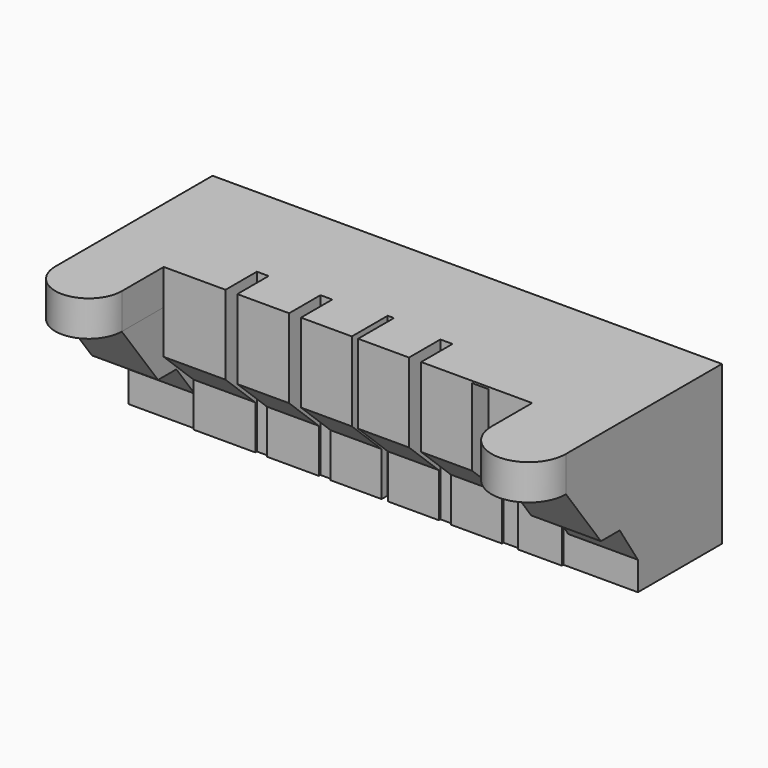
from build123d import *

# Parameters (mm, degrees)
F0_W      = 154.4681414962
F0_H      = 32.4599891901
F1_DEPTH  = 48.0146426708
F2_W      = 11.2775340676
F2_H      = 24.0073213354
F3_DEPTH  = 154.6795647591
F4_W      = 20.4018931836
F4_H      = 24.0073213354
F4_W_2    = 3.5617277026
F4_W_3    = 3.5835206509
F4_W_4    = 3.6845356226
F4_W_5    = 4.9127191305
F4_W_6    = 22.562906146
F4_H_2    = 23.4004920349
F5_DEPTH  = 11.8805598468
F7_DEPTH  = 10.7736643404
F9_DEPTH  = 20.0494788587
F11_DEPTH = 21.1268346757
F12_W     = 1.8992722034
F12_H     = 24.0073213354
F13_DEPTH = 13.5909728706


with BuildPart() as f1:
    # F0 (on Top) → F1 (new body)
    with BuildSketch(Plane.XY):
        with Locations((3.7253e-06, -0.5876496434)):
            Rectangle(F0_W, F0_H)
    extrude(amount=F1_DEPTH)

    # F2 (on face) → F3 (join)
    with BuildSketch(Plane.YZ.offset(77.2340744734)):
        with Locations((-22.4564112723, 36.0109820031)):
            Rectangle(F2_W, F2_H)
        Polygon((-16.8176442385, 13.3598086642), (-16.8176442385, 24.0073213354), (-28.0951783061, 24.0073213354), align=None)
    extrude(amount=-F3_DEPTH)

    # F4 (on face) → F5 (cut)
    with BuildSketch(Plane.XZ.offset(28.0951783061)):
        with Locations((-67.244543694, 12.0036606677)):
            Rectangle(F4_W, F4_H)
        with Locations((-67.244543694, 36.0109820031)):
            Rectangle(F4_W, F4_H)
        with Locations((-36.5212969482, 12.0036606677)):
            Rectangle(F4_W_2, F4_H)
        with Locations((-36.5212969482, 36.0109820031)):
            Rectangle(F4_W_2, F4_H)
        with Locations((-17.2269493341, 36.0109820031)):
            Rectangle(F4_W_3, F4_H)
        with Locations((-17.2269493341, 12.0036606677)):
            Rectangle(F4_W_3, F4_H)
        with Locations((19.1767290235, 36.0109820031)):
            Rectangle(F4_W_4, F4_H)
        with Locations((19.1767290235, 12.0036606677)):
            Rectangle(F4_W_4, F4_H)
        with Locations((38.9504507184, 12.0036606677)):
            Rectangle(F4_W_5, F4_H)
        with Locations((65.9526214004, 36.0109820031)):
            Rectangle(F4_W_6, F4_H)
        with Locations((65.9526214004, 12.0036606677)):
            Rectangle(F4_W_6, F4_H)
        with Locations((38.9504507184, 35.7075673528)):
            Rectangle(F4_W_5, F4_H_2)
    extrude(amount=-F5_DEPTH, mode=Mode.SUBTRACT)

    # F6 (on face) → F7 (join)
    with BuildSketch(Plane.XY.offset(48.0146426708)):
        Polygon((-57.0435971022, -16.2146184593), (-77.2340670228, -16.2146184593), (-77.2340670228, -43.9355224371), (-57.0435971022, -43.9355224371), (-57.0435971022, -28.0951783061), align=None)
        with BuildLine():
            Line((-57.0435971022, -43.9355224371), (-77.2340670228, -43.9355224371))
            ThreePointArc((-77.2340670228, -43.9355224371), (-67.1388320625, -54.0307573974), (-57.0435971022, -43.9355224371))
        make_face()
        Polygon((77.2340744734, -43.4713661671), (77.2340744734, -16.2146184593), (54.6711683273, -16.2146184593), (54.6711683273, -28.0951783061), (54.6711683273, -43.4713661671), align=None)
        with BuildLine():
            ThreePointArc((54.6711683273, -43.4713661671), (65.9526214004, -54.7528192401), (77.2340744734, -43.4713661671))
            Line((77.2340744734, -43.4713661671), (54.6711683273, -43.4713661671))
        make_face()
    extrude(amount=-F7_DEPTH)

    # F8 (on face) → F9 (join)
    with BuildSketch(Plane(origin=(-77.2340670228, 0, 0), x_dir=(0, -1, 0), z_dir=(-1, 0, 0))):
        Polygon((30.0750704482, 18.6204891652), (43.9355224371, 37.2409783304), (16.2146184593, 37.2409783304), (16.2146184593, 18.6204891652), (23.1448444538, 18.6204891652), align=None)
        Polygon((16.2146184593, 9.3102445826), (23.1448444538, 18.6204891652), (16.2146184593, 18.6204891652), align=None)
    extrude(amount=-F9_DEPTH)

    # F10 (on face) → F11 (join)
    with BuildSketch(Plane.YZ.offset(77.2340744734)):
        Polygon((-16.2146184593, 37.2409783304), (-43.4713661671, 37.2409783304), (-30.2190445364, 19.3241238594), (-23.1028571725, 19.3241238594), (-16.2146184593, 8.6756854873), align=None)
    extrude(amount=-F11_DEPTH)

    # F12 (on face) → F13 (cut)
    with BuildSketch(Plane.XZ.offset(28.0951783061)):
        with Locations((0.9496361017, 36.0109820031)):
            Rectangle(F12_W, F12_H)
        with Locations((0.9496361017, 12.0036606677)):
            Rectangle(F12_W, F12_H)
    extrude(amount=-F13_DEPTH, mode=Mode.SUBTRACT)


solid = f1.part
